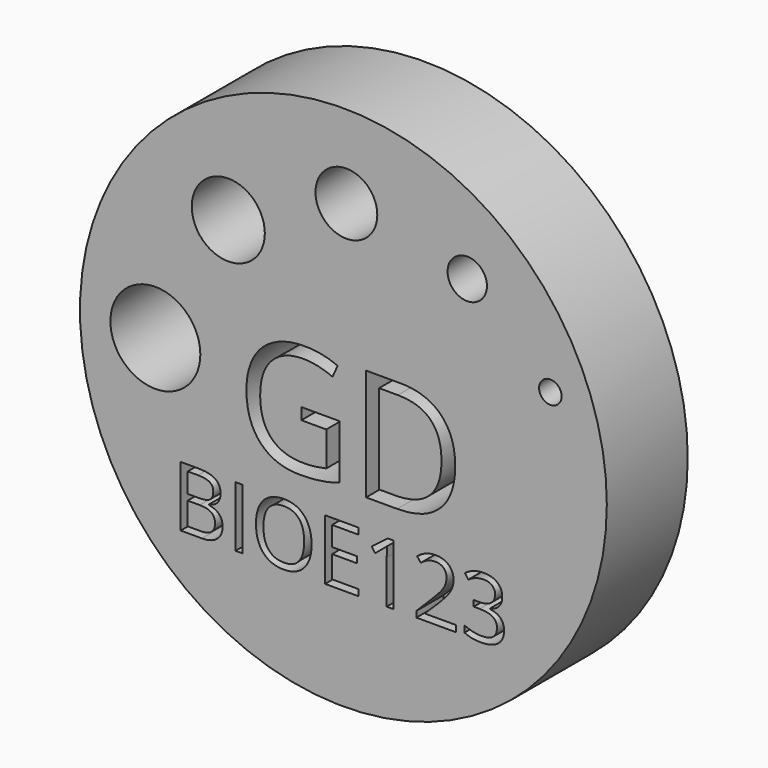
from build123d import *

# Parameters (mm, degrees)
F0_R         = 23.4365
F1_DEPTH     = 9
F2_R         = 4
F2_R_2       = 3.25
F2_R_3       = 2.75
F2_R_4       = 1.75
F2_R_5       = 1
F3_DEPTH     = 9
F4_TEXT_SIZE = 13.9151045762
F5_DEPTH     = 9
F6_TEXT_SIZE = 7.5320701424
F7_DEPTH     = 3


# Not quite as in the source:
# - Text() gives the source's letters only with a copy of the font that has no kerning and outlines rounded to 1/6400 em; it was checked with that copy


with BuildPart() as f1:
    # F0 (on Front) → F1 (new body)
    with BuildSketch(Plane.XZ):
        Circle(F0_R)
    extrude(amount=-F1_DEPTH)

    # F2 (on Front) → F3 (cut)
    with BuildSketch(Plane.XZ):
        with Locations((-16.7306032029, 0)):
            Circle(F2_R)
        with Locations((-10.2427472395, 11.3465488841)):
            Circle(F2_R_2)
        with Locations((0.264364346, 16.0439414204)):
            Circle(F2_R_3)
        with Locations((11.017489247, 13.6466622353)):
            Circle(F2_R_4)
        with Locations((18.4116128074, 7.1751135777)):
            Circle(F2_R_5)
    extrude(amount=-F3_DEPTH, mode=Mode.SUBTRACT)

    # F4 (on Front) → F5 (cut)
    with BuildSketch(Plane.XZ):
        with Locations((-9.4781167936, -6.3999089288)):
            Text('GD', F4_TEXT_SIZE, font='Open Sans', text_align=(TextAlign.LEFT, TextAlign.BOTTOM))
    extrude(amount=-F5_DEPTH, mode=Mode.SUBTRACT)

    # F6 (on Front) → F7 (cut)
    with BuildSketch(Plane.XZ):
        with Locations((-15.2175587005, -14.3600630259)):
            Text('BIOE123', F6_TEXT_SIZE, font='Open Sans', text_align=(TextAlign.LEFT, TextAlign.BOTTOM))
    extrude(amount=-F7_DEPTH, mode=Mode.SUBTRACT)


solid = f1.part
